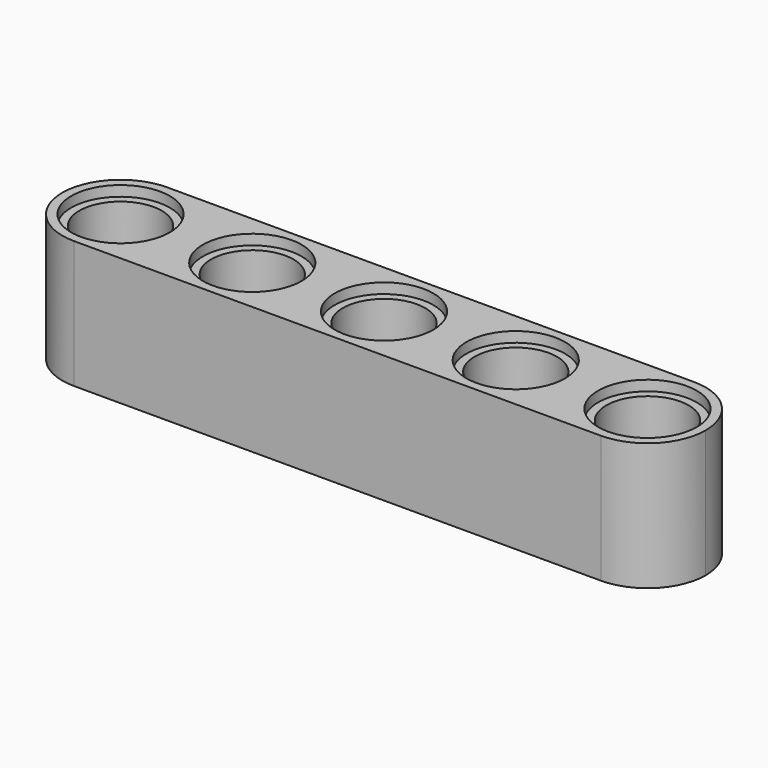
from build123d import *

# Parameters (mm, degrees)
F0_R     = 3.048
F0_R_2   = 2.54
F1_DEPTH = 3.937
F2_R     = 3.0417071759
F3_DEPTH = 0.635
F4_R     = 3.048
F5_DEPTH = 0.635
F6_SIZE2 = 0.50799
F6_SIZE  = 0.50799
F7_SIZE2 = 0.50799
F7_SIZE  = 0.50799


# Not quite as in the source:
# - a fillet or chamfer is up to 0.001 mm smaller than in the source, because OpenCascade refuses the exact size


with BuildPart() as f1:
    # F0 (on Top) → F1 (new body, symmetric)
    with BuildSketch(Plane.XY):
        with BuildLine():
            ThreePointArc((-40.9946195992, 14.3710068385), (-42.0464330806, 16.9103092103), (-44.5857354524, 17.9621226917))
            ThreePointArc((-44.5857354524, 17.9621226917), (-48.1768513056, 14.3710068385), (-44.5857354524, 10.7798909853))
            ThreePointArc((-44.5857354524, 10.7798909853), (-42.0464330806, 11.8317044667), (-40.9946195992, 14.3710068385))
        make_face()
        with Locations((-44.5857354524, 14.3710068385)):
            Circle(F0_R, mode=Mode.SUBTRACT)
        with BuildLine():
            ThreePointArc((-49.1226195992, 14.3710068385), (-50.1744330806, 16.9103092103), (-52.7137354524, 17.9621226917))
            ThreePointArc((-52.7137354524, 17.9621226917), (-56.3048513056, 14.3710068385), (-52.7137354524, 10.7798909853))
            ThreePointArc((-52.7137354524, 10.7798909853), (-50.1744330806, 11.8317044667), (-49.1226195992, 14.3710068385))
        make_face()
        with Locations((-52.7137354524, 14.3710068385)):
            Circle(F0_R, mode=Mode.SUBTRACT)
        with BuildLine():
            ThreePointArc((-32.8666195992, 14.3710068385), (-33.9184330806, 16.9103092103), (-36.4577354524, 17.9621226917))
            ThreePointArc((-36.4577354524, 17.9621226917), (-40.0488513056, 14.3710068385), (-36.4577354524, 10.7798909853))
            ThreePointArc((-36.4577354524, 10.7798909853), (-33.9184330806, 11.8317044667), (-32.8666195992, 14.3710068385))
        make_face()
        with Locations((-36.4577354524, 14.3710068385)):
            Circle(F0_R, mode=Mode.SUBTRACT)
        with BuildLine():
            ThreePointArc((-24.7386195992, 14.3710068385), (-25.7904330806, 16.9103092103), (-28.3297354524, 17.9621226917))
            ThreePointArc((-28.3297354524, 17.9621226917), (-31.9208513056, 14.3710068385), (-28.3297354524, 10.7798909853))
            ThreePointArc((-28.3297354524, 10.7798909853), (-25.7904330806, 11.8317044667), (-24.7386195992, 14.3710068385))
        make_face()
        with Locations((-28.3297354524, 14.3710068385)):
            Circle(F0_R, mode=Mode.SUBTRACT)
        with BuildLine():
            ThreePointArc((-60.8417354524, 10.7798909853), (-58.3024330806, 11.8317044667), (-57.2506195992, 14.3710068385))
            ThreePointArc((-57.2506195992, 14.3710068385), (-58.3024330806, 16.9103092103), (-60.8417354524, 17.9621226917))
            ThreePointArc((-60.8417354524, 17.9621226917), (-64.4328513056, 14.3710068385), (-60.8417354524, 10.7798909853))
        make_face()
        with Locations((-60.8417354524, 14.3710068385)):
            Circle(F0_R, mode=Mode.SUBTRACT)
        with Locations((-44.5857354524, 14.3710068385)):
            Circle(F0_R)
        with Locations((-44.5857354524, 14.3710068385)):
            Circle(F0_R_2, mode=Mode.SUBTRACT)
        with Locations((-36.4577354524, 14.3710068385)):
            Circle(F0_R)
        with Locations((-36.4577354524, 14.3710068385)):
            Circle(F0_R_2, mode=Mode.SUBTRACT)
        with Locations((-52.7137354524, 14.3710068385)):
            Circle(F0_R)
        with Locations((-52.7137354524, 14.3710068385)):
            Circle(F0_R_2, mode=Mode.SUBTRACT)
        with Locations((-28.3297354524, 14.3710068385)):
            Circle(F0_R)
        with Locations((-28.3297354524, 14.3710068385)):
            Circle(F0_R_2, mode=Mode.SUBTRACT)
        with Locations((-60.8417354524, 14.3710068385)):
            Circle(F0_R)
        with Locations((-60.8417354524, 14.3710068385)):
            Circle(F0_R_2, mode=Mode.SUBTRACT)
        with BuildLine():
            ThreePointArc((-60.8417354524, 17.9621226917), (-58.3024330806, 16.9103092103), (-57.2506195992, 14.3710068385))
            ThreePointArc((-57.2506195992, 14.3710068385), (-58.3024330806, 11.8317044667), (-60.8417354524, 10.7798909853))
            Line((-60.8417354524, 10.7798909853), (-52.7137354524, 10.7798909853))
            ThreePointArc((-52.7137354524, 10.7798909853), (-56.3048513056, 14.3710068385), (-52.7137354524, 17.9621226917))
            Line((-52.7137354524, 17.9621226917), (-60.8417354524, 17.9621226917))
        make_face()
        with BuildLine():
            Line((-44.5857354524, 17.9621226917), (-52.7137354524, 17.9621226917))
            ThreePointArc((-52.7137354524, 17.9621226917), (-50.1744330806, 16.9103092103), (-49.1226195992, 14.3710068385))
            ThreePointArc((-49.1226195992, 14.3710068385), (-50.1744330806, 11.8317044667), (-52.7137354524, 10.7798909853))
            Line((-52.7137354524, 10.7798909853), (-44.5857354524, 10.7798909853))
            ThreePointArc((-44.5857354524, 10.7798909853), (-48.1768513056, 14.3710068385), (-44.5857354524, 17.9621226917))
        make_face()
        with BuildLine():
            Line((-28.3297354524, 17.9621226917), (-36.4577354524, 17.9621226917))
            ThreePointArc((-36.4577354524, 17.9621226917), (-33.9184330806, 16.9103092103), (-32.8666195992, 14.3710068385))
            ThreePointArc((-32.8666195992, 14.3710068385), (-33.9184330806, 11.8317044667), (-36.4577354524, 10.7798909853))
            Line((-36.4577354524, 10.7798909853), (-28.3297354524, 10.7798909853))
            ThreePointArc((-28.3297354524, 10.7798909853), (-31.9208513056, 14.3710068385), (-28.3297354524, 17.9621226917))
        make_face()
        with BuildLine():
            Line((-36.4577354524, 17.9621226917), (-44.5857354524, 17.9621226917))
            ThreePointArc((-44.5857354524, 17.9621226917), (-42.0464330806, 16.9103092103), (-40.9946195992, 14.3710068385))
            ThreePointArc((-40.9946195992, 14.3710068385), (-42.0464330806, 11.8317044667), (-44.5857354524, 10.7798909853))
            Line((-44.5857354524, 10.7798909853), (-36.4577354524, 10.7798909853))
            ThreePointArc((-36.4577354524, 10.7798909853), (-40.0488513056, 14.3710068385), (-36.4577354524, 17.9621226917))
        make_face()
    extrude(amount=F1_DEPTH, both=True)

    # F2 (on face) → F3 (cut)
    with BuildSketch(Plane.XY.offset(3.937)):
        with Locations((-28.3297354524, 14.3710068385)):
            Circle(F2_R)
        with Locations((-36.4577354524, 14.3710068385)):
            Circle(F2_R)
        with Locations((-44.5857354524, 14.3710068385)):
            Circle(F2_R)
        with Locations((-52.7137354524, 14.3710068385)):
            Circle(F2_R)
        with Locations((-60.8417354524, 14.3710068385)):
            Circle(F2_R)
    extrude(amount=-F3_DEPTH, mode=Mode.SUBTRACT)

    # F4 (on face) → F5 (cut)
    with BuildSketch(Plane(origin=(0, 0, -3.937), x_dir=(1, 0, 0), z_dir=(0, 0, -1))):
        with Locations((-60.8417354524, -14.3710068385)):
            Circle(F4_R)
        with Locations((-52.7137354524, -14.3710068385)):
            Circle(F4_R)
        with Locations((-44.5857354524, -14.3710068385)):
            Circle(F4_R)
        with Locations((-36.4577354524, -14.3710068385)):
            Circle(F4_R)
        with Locations((-28.3297354524, -14.3710068385)):
            Circle(F4_R)
    extrude(amount=-F5_DEPTH, mode=Mode.SUBTRACT)

    # F6 (size 0.508 and 0.508 in the source; OpenCascade refuses exactly that, so slightly less here)
    f6_edges = [f1.edges().sort_by_distance(p)[0] for p in [
        (-38.997735, 14.371007, -3.302),
    ]]
    chamfer(f6_edges, length=F6_SIZE, length2=F6_SIZE2)

    # F7 (size 0.508 and 0.508 in the source; OpenCascade refuses exactly that, so slightly less here)
    f7_edges = [f1.edges().sort_by_distance(p)[0] for p in [
        (-47.125735, 14.371007, -3.302),
        (-55.253735, 14.371007, -3.302),
        (-63.381735, 14.371007, -3.302),
        (-30.869735, 14.371007, -3.302),
    ]]
    chamfer(f7_edges, length=F7_SIZE, length2=F7_SIZE2)


solid = f1.part
